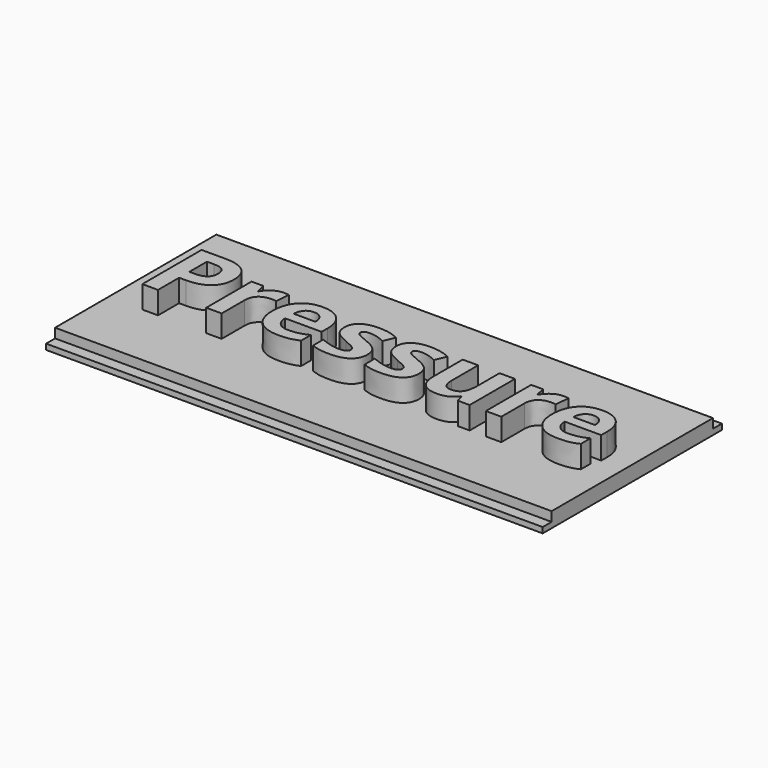
from build123d import *

# Parameters (mm, degrees)
F1_DEPTH     = 13.3
F2_TEXT_SIZE = 5.5555555556
F3_DEPTH     = 1.2


# Not quite as in the source:
# - Text() gives the source's letters only with a copy of the font that has no kerning and outlines rounded to 1/6400 em; it was checked with that copy


with BuildPart() as f1:
    # F0 (on Right) → F1 (new body, symmetric)
    with BuildSketch(Plane.YZ):
        Polygon((-6, -0.15), (6, -0.15), (6, 0.15), (5.4, 0.15), (5.4, 0.6564130308), (-5.4, 0.6564130308), (-5.4, 0.15), (-6, 0.15), align=None)
    extrude(amount=F1_DEPTH, both=True)

    # F2 (on face) → F3 (join)
    with BuildSketch(Plane.XY.offset(0.6564130308)):
        with Locations((-11.9752505003, -1.8368388966)):
            Text('Pressure', F2_TEXT_SIZE, font='Open Sans', font_style=FontStyle.BOLD, text_align=(TextAlign.LEFT, TextAlign.BOTTOM))
    extrude(amount=F3_DEPTH)


solid = f1.part
